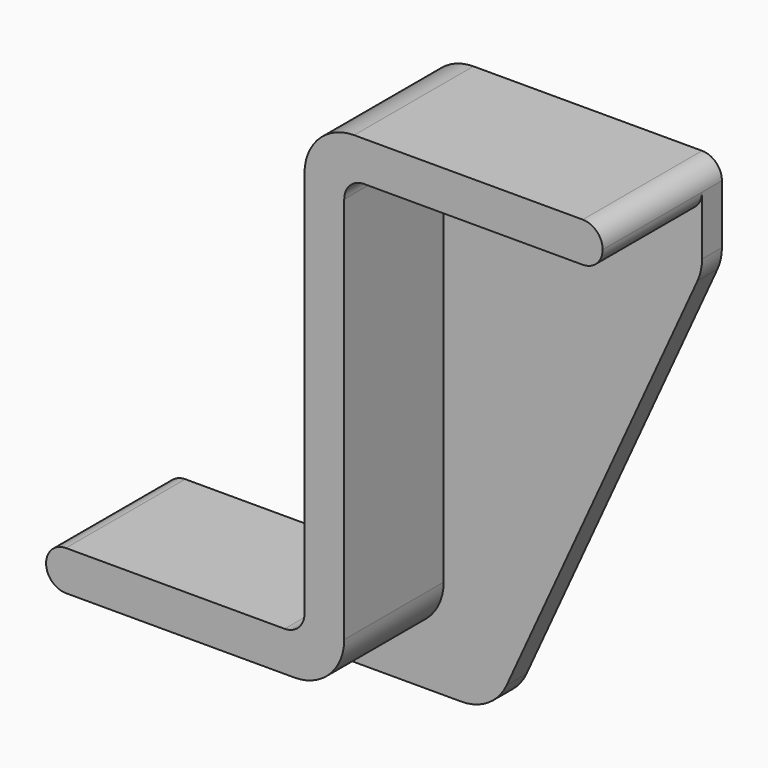
from build123d import *

# Parameters (mm, degrees)
F1_DEPTH = 19.05
F2_DEPTH = 3.175
F3_R     = 6.35
F4_R     = 2.53999
F5_R     = 2.54


# Not quite as in the source:
# - a fillet or chamfer is up to 0.001 mm smaller than in the source, because OpenCascade refuses the exact size


with BuildPart() as f1:
    # F0 (on Front) → F1 (new body)
    with BuildSketch(Plane.XZ):
        Polygon((-33.02, 0), (0, 0), (5.08, 0), (5.08, 5.08), (5.08, 58.42), (38.1, 58.42), (38.1, 63.5), (5.08, 63.5), (0, 63.5), (0, 58.42), (0, 5.08), (-33.02, 5.08), align=None)
    extrude(amount=F1_DEPTH)

    # F0 (on Front) → F2 (join)
    with BuildSketch(Plane.XZ):
        with BuildLine():
            Line((5.08, 0), (0, 0))
            Line((0, 0), (-33.02, 0))
            ThreePointArc((-33.02, 0), (-31.1601280605, -4.4901280605), (-26.67, -6.35))
            Line((-26.67, -6.35), (7.3484978099, -6.35))
            ThreePointArc((7.3484978099, -6.35), (10.7819271621, -5.3417284546), (13.1250166344, -2.6371064199))
            Line((13.1250166344, -2.6371064199), (37.5265188245, 50.8138031394))
            ThreePointArc((37.5265188245, 50.8138031394), (37.9549735912, 52.1015383235), (38.1, 53.4509095593))
            Line((38.1, 53.4509095593), (38.1, 58.42))
            Line((38.1, 58.42), (5.08, 58.42))
            Line((5.08, 58.42), (5.08, 5.08))
            Line((5.08, 5.08), (5.08, 0))
        make_face()
    extrude(amount=F2_DEPTH)

    # F3
    f3_edges = [f1.edges().sort_by_distance(p)[0] for p in [
        (0, -9.525, 63.5),
        (5.08, -11.1125, 0),
    ]]
    fillet(f3_edges, radius=F3_R)

    # F4 (radius 2.54 in the source; OpenCascade refuses exactly that, so slightly less here)
    f4_edges = [f1.edges().sort_by_distance(p)[0] for p in [
        (-33.02, -11.1125, 0),
        (-33.02, -1.5875, 0),
        (-33.02, -9.525, 5.08),
        (38.1, -11.1125, 58.42),
        (38.1, -9.525, 63.5),
    ]]
    fillet(f4_edges, radius=F4_R)

    # F5
    f5_edges = [f1.edges().sort_by_distance(p)[0] for p in [
        (5.08, -11.1125, 58.42),
        (0, -9.525, 5.08),
    ]]
    fillet(f5_edges, radius=F5_R)


solid = f1.part
